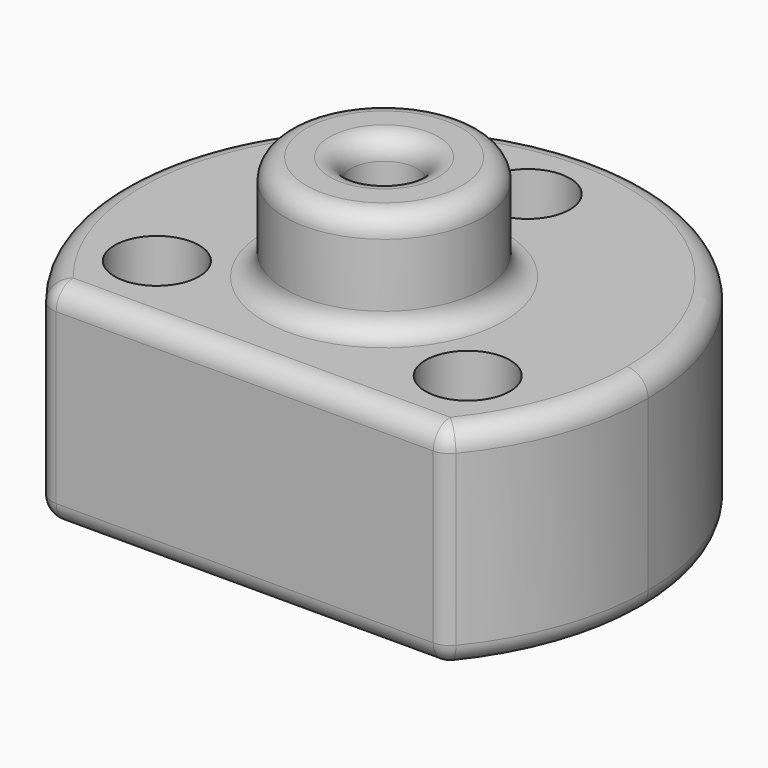
from build123d import *

# Parameters (mm, degrees)
F0_R        = 2
F0_R_2      = 4.682431568
F1_DEPTH    = 10
F0_R_3      = 3.1
F0_R_4      = 1.575
F2_DEPTH    = 15
F1_FACE_R   = 2
F1_FACE_R_2 = 4.682431568
F3_DEPTH    = 3
F5_DEPTH    = 6
F6_R        = 1


with BuildPart() as f1:
    # F0 (on Top) → F1 (new body)
    with BuildSketch(Plane.XY):
        with BuildLine():
            ThreePointArc((9.3908199855, -8.25), (11.6969066385, -4.4082167699), (12.5, 0))
            ThreePointArc((12.5, 0), (-4.4082167699, 11.6969066385), (-9.3908199855, -8.25))
            Line((-9.3908199855, -8.25), (9.3908199855, -8.25))
        make_face()
        with Locations((-7.3612159322, -4.25)):
            Circle(F0_R, mode=Mode.SUBTRACT)
        with Locations((7.3612159322, -4.25)):
            Circle(F0_R, mode=Mode.SUBTRACT)
        Circle(F0_R_2, mode=Mode.SUBTRACT)
        with Locations((0, 8.5)):
            Circle(F0_R, mode=Mode.SUBTRACT)
    extrude(amount=F1_DEPTH)

    # F0 (on Top) → F2 (join)
    with BuildSketch(Plane.XY):
        Circle(F0_R_2)
        Circle(F0_R_3, mode=Mode.SUBTRACT)
        Circle(F0_R_3)
        Circle(F0_R_4, mode=Mode.SUBTRACT)
    extrude(amount=F2_DEPTH)

    # F1_face (on face) + F0 (on Top) → F3 (cut)
    with BuildSketch(Plane(origin=(0, 1.6783251384, 10), x_dir=(1, 0, 0), z_dir=(0, 0, 1))):
        with BuildLine():
            ThreePointArc((9.3908199855, -9.9283251384), (0, 10.8216748616), (-9.3908199855, -9.9283251384))
            Line((-9.3908199855, -9.9283251384), (9.3908199855, -9.9283251384))
        make_face()
        with Locations((-7.3612159322, -5.9283251384)):
            Circle(F1_FACE_R, mode=Mode.SUBTRACT)
        with Locations((7.3612159322, -5.9283251384)):
            Circle(F1_FACE_R, mode=Mode.SUBTRACT)
        with Locations((0, -1.6783251384)):
            Circle(F1_FACE_R_2, mode=Mode.SUBTRACT)
        with Locations((0, 6.8216748616)):
            Circle(F1_FACE_R, mode=Mode.SUBTRACT)
    with BuildSketch(Plane.XY):
        Circle(F0_R_3)
        Circle(F0_R_4, mode=Mode.SUBTRACT)
    extrude(amount=F3_DEPTH, mode=Mode.SUBTRACT)

    # F4 (on Top) → F5 (cut)
    with BuildSketch(Plane.XY):
        Polygon((2.7, -1.5588457268), (2.7, 1.5588457268), (0, 3.1176914536), (-2.7, 1.5588457268), (-2.7, -1.5588457268), (0, -3.1176914536), align=None)
    extrude(amount=F5_DEPTH, mode=Mode.SUBTRACT)

    # F6
    f6_edges = [f1.edges().sort_by_distance(p)[0] for p in [
        (-1.575, 0, 15),
        (-4.682432, 0, 15),
        (-4.682432, 0, 10),
        (0, 12.5, 10),
        (0, -8.25, 10),
        (0, 12.5, 0),
        (0, -8.25, 0),
        (9.39082, -8.25, 5),
        (-9.39082, -8.25, 5),
    ]]
    fillet(f6_edges, radius=F6_R)


solid = f1.part
